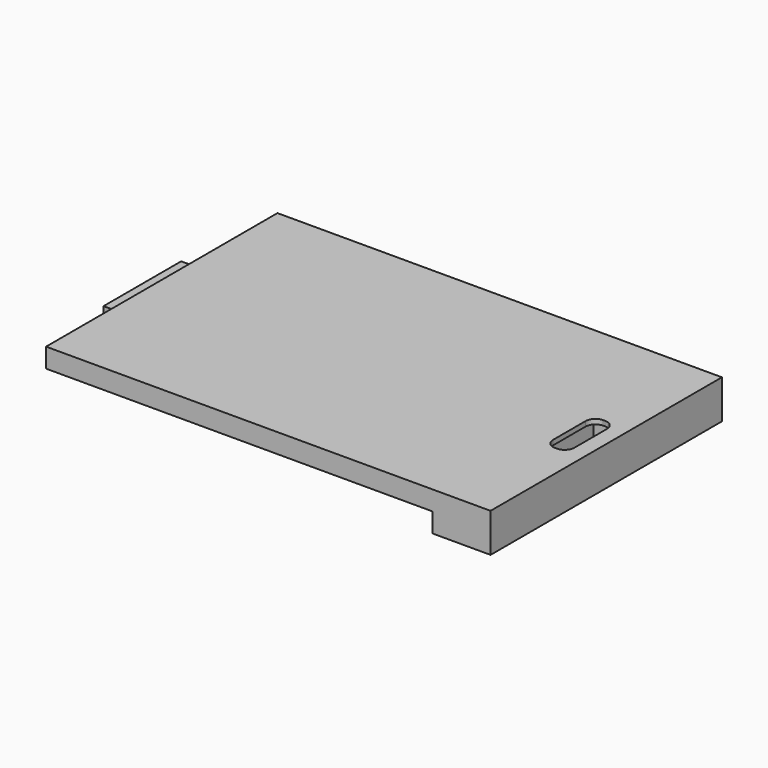
from build123d import *

# Parameters (mm, degrees)
F0_W        = 58.166
F0_H        = 37.846
F1_DEPTH    = 2.54
F2_W        = 7.5946
F2_H        = 37.846
F3_DEPTH    = 2.54
F4_W        = 12.7
F4_H        = 0.635
F4_H_2      = 1.27
F5_DEPTH    = 2.54
F6_T1_DEPTH = 12.7
F7_W        = 4.445
F7_H        = 10.16
F8_DEPTH    = 4.445
F9_W        = 4.445
F9_H        = 5.08
F10_DEPTH   = 0.635
F12_DEPTH   = 0.635
F13_W       = 6.35
F13_H       = 6.35
F14_DEPTH   = 2.794


# Not quite as in the source:
# - a fillet or chamfer that OpenCascade refuses, or shapes differently, is made with other operations: its cross-section is extruded or revolved along the edge and cut away or added


with BuildPart() as f1:
    # F0 (on Top) → F1 (new body)
    with BuildSketch(Plane.XY):
        Rectangle(F0_W, F0_H)
    extrude(amount=F1_DEPTH)

    # F2 (on face) → F3 (join)
    with BuildSketch(Plane(origin=(0, 0, 0), x_dir=(1, 0, 0), z_dir=(0, 0, -1))):
        with Locations((25.2857, 0)):
            Rectangle(F2_W, F2_H)
    extrude(amount=F3_DEPTH)

    # F4 (on face) → F5 (join)
    with BuildSketch(Plane(origin=(-29.083, 0, 0), x_dir=(0, -1, 0), z_dir=(-1, 0, 0))):
        with Locations((0, -0.3175)):
            Rectangle(F4_W, F4_H)
        with Locations((0, 0.635)):
            Rectangle(F4_W, F4_H_2)
    extrude(amount=F5_DEPTH)

    # F6: fillet of radius 1.27 on 1 edges, made by hand

    # F6_s2 → F6_t1 (join)
    with BuildSketch(Plane.XZ.offset(-6.35)):
        with BuildLine():
            ThreePointArc((-27.9831477372, 0), (-28.6181477372, -0.1701477372), (-29.083, -0.635))
            Line((-29.083, -0.635), (-29.083, 0))
            Line((-29.083, 0), (-27.9831477372, 0))
        make_face()
    extrude(amount=F6_T1_DEPTH)

    # F7 (on face) → F8 (cut)
    with BuildSketch(Plane(origin=(0, 0, -2.54), x_dir=(1, 0, 0), z_dir=(0, 0, -1))):
        with Locations((25.5905, 0)):
            Rectangle(F7_W, F7_H)
    extrude(amount=-F8_DEPTH, mode=Mode.SUBTRACT)

    # F9 (on face) → F10 (cut)
    with BuildSketch(Plane(origin=(0, 0, -2.54), x_dir=(1, 0, 0), z_dir=(0, 0, -1))):
        with Locations((25.5905, 7.62)):
            Rectangle(F9_W, F9_H)
    extrude(amount=-F10_DEPTH, mode=Mode.SUBTRACT)

    # F11 (on face) → F12 (cut, through all)
    with BuildSketch(Plane(origin=(0, 0, 1.905), x_dir=(1, 0, 0), z_dir=(0, 0, -1))):
        with BuildLine():
            Line((25.527, -3.937), (25.781, -3.937))
            ThreePointArc((25.781, -3.937), (26.6790256121, -3.5650256121), (27.051, -2.667))
            Line((27.051, -2.667), (27.051, 2.667))
            ThreePointArc((27.051, 2.667), (26.6790256121, 3.5650256121), (25.781, 3.937))
            Line((25.781, 3.937), (25.527, 3.937))
            ThreePointArc((25.527, 3.937), (24.6289743879, 3.5650256121), (24.257, 2.667))
            Line((24.257, 2.667), (24.257, -2.667))
            ThreePointArc((24.257, -2.667), (24.6289743879, -3.5650256121), (25.527, -3.937))
        make_face()
    extrude(amount=-F12_DEPTH, mode=Mode.SUBTRACT)

    # F13 (on face) → F14 (cut)
    with BuildSketch(Plane(origin=(0, 0, -2.54), x_dir=(1, 0, 0), z_dir=(0, 0, -1))):
        with Locations((25.273, 15.113)):
            Rectangle(F13_W, F13_H)
    extrude(amount=-F14_DEPTH, mode=Mode.SUBTRACT)


solid = f1.part
